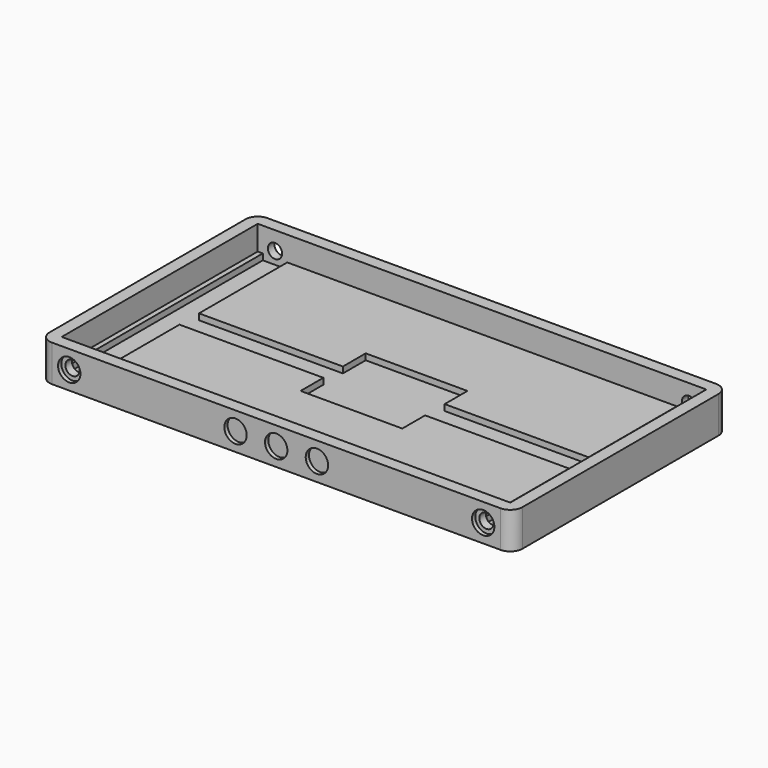
from build123d import *

# Parameters (mm, degrees)
F0_W     = 110.2
F0_H     = 60.2
F1_DEPTH = 3
F0_W_2   = 116.2
F0_H_2   = 66.2
F2_DEPTH = 9
F3_W     = 35.35
F3_H     = 6
F4_DEPTH = 1.5
F5_R     = 1.75
F6_DEPTH = 25
F5_R_2   = 2.75
F7_DEPTH = 1
F8_R     = 3


# Not quite as in the source:
# - a pattern or mirror of a feature is missing from the dataset's text; its kind, count and spacing are read off the source's solid


with BuildPart() as f1:
    # F0 (on Top) → F1 (new body)
    with BuildSketch(Plane.XY):
        Rectangle(F0_W, F0_H)
    extrude(amount=F1_DEPTH)

    # F0 (on Top) → F2 (join)
    with BuildSketch(Plane.XY):
        Rectangle(F0_W_2, F0_H_2)
        Rectangle(F0_W, F0_H, mode=Mode.SUBTRACT)
    extrude(amount=F2_DEPTH)

    # F3 (on face) → F4 (cut)
    with BuildSketch(Plane.XY.offset(3)):
        Polygon((-12.5, 10), (-12.5, 3), (-12.5, -3), (-12.5, -10), (12.5, -10), (12.5, -3), (12.5, 3), (12.5, 10), align=None)
        with Locations((-30.175, 0)):
            Rectangle(F3_W, F3_H)
        with Locations((30.175, 0)):
            Rectangle(F3_W, F3_H)
        Polygon((-47.85, 30.1), (-53.85, 30.1), (-53.85, -30.1), (-47.85, -30.1), (-47.85, -3), (-47.85, 3), align=None)
        Polygon((53.85, 30.1), (47.85, 30.1), (47.85, 3), (47.85, -3), (47.85, -30.1), (53.85, -30.1), align=None)
    extrude(amount=-F4_DEPTH, mode=Mode.SUBTRACT)

    # F5 (on face) → F6 (cut)
    with BuildSketch(Plane.XZ.offset(33.1)):
        with Locations((-50.85, 4.5)):
            Circle(F5_R)
        with Locations((50.85, 4.5)):
            Circle(F5_R)
    f6 = extrude(amount=-F6_DEPTH, mode=Mode.SUBTRACT)

    # F6_copies: F6 across plane
    add(f6.mirror(Plane.ZX), mode=Mode.SUBTRACT)

    # F5 (on face) → F7 (cut)
    with BuildSketch(Plane.XZ.offset(33.1)):
        with Locations((-50.85, 4.5)):
            Circle(F5_R_2)
        with Locations((-50.85, 4.5)):
            Circle(F5_R, mode=Mode.SUBTRACT)
        with Locations((-10, 4.5)):
            Circle(F5_R_2)
        with Locations((0, 4.5)):
            Circle(F5_R_2)
        with Locations((10, 4.5)):
            Circle(F5_R_2)
        with Locations((50.85, 4.5)):
            Circle(F5_R_2)
        with Locations((50.85, 4.5)):
            Circle(F5_R, mode=Mode.SUBTRACT)
    f7 = extrude(amount=-F7_DEPTH, mode=Mode.SUBTRACT)

    # F7_copies: F7 across plane
    add(f7.mirror(Plane.ZX), mode=Mode.SUBTRACT)

    # F8
    f8_edges = [f1.edges().sort_by_distance(p)[0] for p in [
        (58.1, -33.1, 4.5),
        (-58.1, -33.1, 4.5),
        (58.1, 33.1, 4.5),
        (-58.1, 33.1, 4.5),
    ]]
    fillet(f8_edges, radius=F8_R)


solid = f1.part
